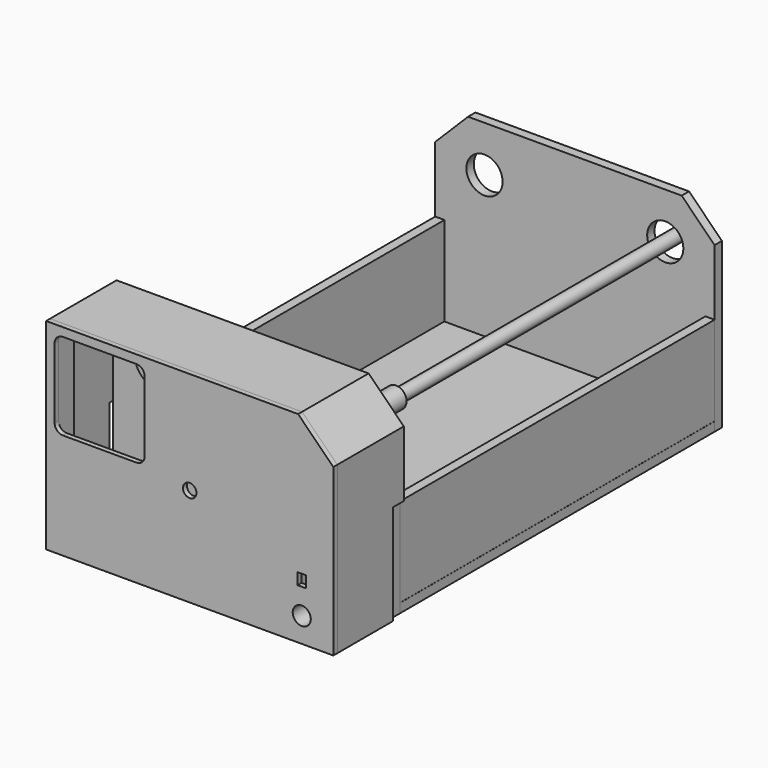
from build123d import *

# Parameters (mm, degrees)
F0_W      = 170
F0_H      = 120
F0_R      = 11
F1_DEPTH  = 5.6
F2_SIZE   = 20
F4_W      = 170
F4_H      = 239.4
F5_DEPTH  = 5.6
F7_W      = 239.4
F7_H      = 54.3528907001
F8_DEPTH  = 5.6
F11_R     = 5.5
F11_R_2   = 4
F12_DEPTH = 25
F13_R     = 1.6
F13_R_2   = 11
F13_R_3   = 6
F14_DEPTH = 3
F15_R     = 3.925
F16_DEPTH = 135
F18_R     = 6.4
F18_R_2   = 4
F19_DEPTH = 34.1
F22_DEPTH = 5.6
F23_DEPTH = 45
F25_DEPTH = 45
F26_W     = 8.2
F26_H     = 61
F27_DEPTH = 25
F28_W     = 8.2
F28_H     = 61
F29_DEPTH = 25
F31_DEPTH = 12
F33_DEPTH = 3
F34_W     = 54.8
F34_H     = 52.8
F35_DEPTH = 25
F36_R     = 5
F37_W     = 5
F37_H     = 7
F37_R     = 4.1
F37_R_2   = 5.5
F38_DEPTH = 25
F39_W     = 12.2999991775
F39_H     = 19.7999991775
F39_W_2   = 7.5
F39_H_2   = 15
F40_DEPTH = 8
F41_R     = 7.8999982774
F41_R_2   = 5.5
F42_DEPTH = 8
F43_W     = 164.7
F43_H     = 2.4
F44_DEPTH = 42
F45_DEPTH = 2.4
F46_DEPTH = 2.4
F47_W     = 2.4
F47_H     = 30
F48_DEPTH = 10


with BuildPart() as f1:
    # F0 (on Front) → F1 (new body)
    with BuildSketch(Plane.XZ):
        Rectangle(F0_W, F0_H)
        with Locations((-55, 32)):
            Circle(F0_R, mode=Mode.SUBTRACT)
        with Locations((55, 32)):
            Circle(F0_R, mode=Mode.SUBTRACT)
    extrude(amount=F1_DEPTH)

    # F2
    f2_edges = [f1.edges().sort_by_distance(p)[0] for p in [
        (-85, -2.8, 60),
        (85, -2.8, 60),
    ]]
    chamfer(f2_edges, length=F2_SIZE)


with BuildPart() as f3_1:
    # F3: copy of F1
    add(f1.part.moved(Location((0, 245, 0))))


with BuildPart() as f5:
    # F4 (on Top) → F5 (new body)
    with BuildSketch(Plane.XY):
        with Locations((0, 119.7)):
            Rectangle(F4_W, F4_H)
    extrude(amount=F5_DEPTH)


with BuildPart() as f5_1:
    # F6: moved
    add(f5.part.moved(Location((0, 0, -60))))


with BuildPart() as f8:
    # F7 (on Right) → F8 (new body)
    with BuildSketch(Plane.YZ):
        with Locations((119.7, -27.1764453501)):
            Rectangle(F7_W, F7_H)
    extrude(amount=F8_DEPTH)


with BuildPart() as f8_1:
    # F9: moved
    add(f8.part.moved(Location((-85, 0, 0))))


with BuildPart() as f10_1:
    # F10: copy of F8
    add(f8_1.part.moved(Location((164.4, 0, 0))))


with BuildPart() as f1_1:
    add(f1.part)

    # F11 (on face) → F12 (cut)
    with BuildSketch(Plane(origin=(0, 0, 0), x_dir=(-1, 0, 0), z_dir=(0, 1, 0))):
        with Locations((0, -36.7425866425)):
            Circle(F11_R)
        with Locations((0, -16.9015619904)):
            Circle(F11_R_2)
    extrude(amount=-F12_DEPTH, mode=Mode.SUBTRACT)


with BuildPart() as f14:
    # F13 (on face) → F14 (new body)
    with BuildSketch(Plane.XZ.offset(5.6)):
        with BuildLine():
            Line((-72.4788332323, 27.5000497816), (-68.7840650039, 27.5000497816))
            ThreePointArc((-68.7840650039, 27.5000497816), (-54.9999830979, 17.5), (-41.2159245053, 27.5000819167))
            Line((-41.2159245053, 27.5000819167), (-37.5271522255, 27.5000819167))
            ThreePointArc((-37.5271522255, 27.5000819167), (-33.000385331, 31.9411117145), (-37.4093785838, 36.4990874362))
            Line((-37.4093785838, 36.4990874362), (-41.2410833772, 36.576266313))
            ThreePointArc((-41.2410833772, 36.576266313), (-55.0427702953, 46.4999369206), (-68.7856740857, 36.4950183541))
            Line((-68.7856740857, 36.4950183541), (-72.2883162832, 36.4950183541))
            Line((-72.2883162832, 36.4950183541), (-72.7116837168, 36.4950183541))
            ThreePointArc((-72.7116837168, 36.4950183541), (-76.998492979, 31.883548646), (-72.4788332323, 27.5000497816))
        make_face()
        with Locations((-72.5, 32)):
            Circle(F13_R, mode=Mode.SUBTRACT)
        with Locations((-55, 32)):
            Circle(F13_R_2, mode=Mode.SUBTRACT)
        with Locations((-37.5, 32)):
            Circle(F13_R, mode=Mode.SUBTRACT)
        with Locations((-55, 32)):
            Circle(F13_R_2)
        with Locations((-55, 32)):
            Circle(F13_R_3, mode=Mode.SUBTRACT)
    extrude(amount=F14_DEPTH)


with BuildPart() as f16:
    # F15 (on Front) → F16 (new body, symmetric)
    with BuildSketch(Plane.XZ):
        with Locations((55.2735887468, 32.0943407714)):
            Circle(F15_R)
    extrude(amount=F16_DEPTH, both=True)


with BuildPart() as f16_1:
    # F17: moved
    add(f16.part.moved(Location((0, 120, 0))))


with BuildPart() as f19:
    # F18 (on face) → F19 (new body)
    with BuildSketch(Plane.XZ.offset(15)):
        with Locations((55.2735887468, 32.0943407714)):
            Circle(F18_R)
        with Locations((55.2735887468, 32.0943407714)):
            Circle(F18_R_2, mode=Mode.SUBTRACT)
    extrude(amount=F19_DEPTH)


with BuildPart() as f19_1:
    # F20: moved
    add(f19.part.moved(Location((0, 49.3, 0))))


with BuildPart() as f22:
    # F21 (on face) → F22 (new body)
    with BuildSketch(Plane.XZ.offset(5.6)):
        Polygon((-87.3999983072, 62.3999983072), (-87.3999983072, 40.9941118485), (-87.3999983072, -60), (-85, -60), (-85, 40), (-65, 60), (65, 60), (85, 40), (85, -60), (87.3999983072, -60), (87.3999983072, 40.9941118485), (65.9941118485, 62.3999983072), (-65.9941118485, 62.3999983072), align=None)
    extrude(amount=-F22_DEPTH)

    # F23 (add): a face of the model
    f23_faces = [f22.faces().sort_by_distance(p)[0] for p in [
        (-85.2660630129, -5.6, 1.1999991536),
    ]]
    extrude(f23_faces, amount=F23_DEPTH)

    # F24 (on face) → F25 (cut)
    with BuildSketch(Plane.XZ.offset(50.6)):
        Polygon((-85, 40), (-65, 60), (-85, 60), align=None)
    extrude(amount=-F25_DEPTH, mode=Mode.SUBTRACT)

    # F26 (on face) → F27 (cut)
    with BuildSketch(Plane(origin=(-87.3999983072, 0, 0), x_dir=(0, -1, 0), z_dir=(-1, 0, 0))):
        with Locations((4.1, -29.5)):
            Rectangle(F26_W, F26_H)
    extrude(amount=-F27_DEPTH, mode=Mode.SUBTRACT)

    # F28 (on face) → F29 (cut)
    with BuildSketch(Plane.YZ.offset(87.3999983072)):
        with Locations((-4.1, -29.5)):
            Rectangle(F28_W, F28_H)
    extrude(amount=-F29_DEPTH, mode=Mode.SUBTRACT)


with BuildPart() as f31:
    # F30 (on face) → F31 (new body)
    with BuildSketch(Plane.XZ.offset(50.6)):
        Polygon((64.8964466094, 59.75), (-84.75, 59.75), (-84.75, -60), (-82.35, -60), (-82.35, 57.35), (63.9023340597, 57.35), (82.35, 38.9023340597), (82.35, -60), (84.75, -60), (84.75, 39.8964466094), align=None)
    extrude(amount=-F31_DEPTH)

    # F32 (on face) → F33 (join)
    with BuildSketch(Plane.XZ.offset(50.6)):
        Polygon((-82.35, 57.35), (-82.35, -60), (82.35, -60), (82.35, 38.9023340597), (63.9023340597, 57.35), align=None)
        Polygon((-84.75, 59.75), (-84.75, -60), (-82.35, -60), (-82.35, 57.35), (63.9023340597, 57.35), (82.35, 38.9023340597), (82.35, -60), (84.75, -60), (84.75, 39.8964466094), (64.8964466094, 59.75), align=None)
        Polygon((87.3999983072, 40.9941118485), (65.9941118485, 62.3999983072), (-87.3999983072, 62.3999983072), (-87.3999983072, -60), (-85, -60), (-84.75, -60), (-84.75, 59.75), (64.8964466094, 59.75), (84.75, 39.8964466094), (84.75, -60), (85, -60), (87.3999983072, -60), align=None)
    extrude(amount=F33_DEPTH)

    # F34 (on face) → F35 (cut)
    with BuildSketch(Plane.XZ.offset(53.6)):
        with Locations((-54.7999983072, 30.7999983072)):
            Rectangle(F34_W, F34_H)
    extrude(amount=-F35_DEPTH, mode=Mode.SUBTRACT)

    # F36
    f36_edges = [f31.edges().sort_by_distance(p)[0] for p in [
        (-27.399998, -52.1, 4.399998),
        (-82.199998, -52.1, 4.399998),
        (-27.399998, -52.1, 57.199998),
        (-82.199998, -52.1, 57.199998),
    ]]
    fillet(f36_edges, radius=F36_R)

    # F37 (on face) → F38 (cut)
    with BuildSketch(Plane.XZ.offset(53.6)):
        with Locations((68.1872093678, -25.89129062)):
            Rectangle(F37_W, F37_H)
        Circle(F37_R)
        with Locations((68.1872093678, -44.9256520867)):
            Circle(F37_R_2)
    extrude(amount=-F38_DEPTH, mode=Mode.SUBTRACT)

    # F39 (on face) → F40 (join)
    with BuildSketch(Plane.XZ.offset(50.6)):
        with Locations((68.1872093678, -25.89129062)):
            Rectangle(F39_W, F39_H)
        with Locations((68.1872093678, -25.89129062)):
            Rectangle(F39_W_2, F39_H_2, mode=Mode.SUBTRACT)
    extrude(amount=-F40_DEPTH)

    # F41 (on face) → F42 (join)
    with BuildSketch(Plane.XZ.offset(50.6)):
        with Locations((68.1872093678, -44.9256520867)):
            Circle(F41_R)
        with Locations((68.1872093678, -44.9256520867)):
            Circle(F41_R_2, mode=Mode.SUBTRACT)
    extrude(amount=-F42_DEPTH)

    # F43 (on face) → F44 (join)
    with BuildSketch(Plane.XZ.offset(50.6)):
        with Locations((0, -58.8)):
            Rectangle(F43_W, F43_H)
    extrude(amount=-F44_DEPTH)

    # F45 (add): a face of the model
    f45_faces = [f31.faces().sort_by_distance(p)[0] for p in [
        (-82.35, -23.6, -58.8),
    ]]
    extrude(f45_faces, amount=F45_DEPTH)

    # F46 (add): a face of the model
    f46_faces = [f31.faces().sort_by_distance(p)[0] for p in [
        (82.35, -23.6, -58.8),
    ]]
    extrude(f46_faces, amount=F46_DEPTH)

    # F47 (on face) → F48 (join)
    with BuildSketch(Plane.XY.offset(-57.6)):
        with Locations((-83.55, -23.6)):
            Rectangle(F47_W, F47_H)
        with Locations((83.55, -23.6)):
            Rectangle(F47_W, F47_H)
    extrude(amount=F48_DEPTH)


solid = Compound([f3_1.part, f5_1.part, f8_1.part, f10_1.part, f1_1.part, f14.part, f16_1.part, f19_1.part, f22.part, f31.part])
